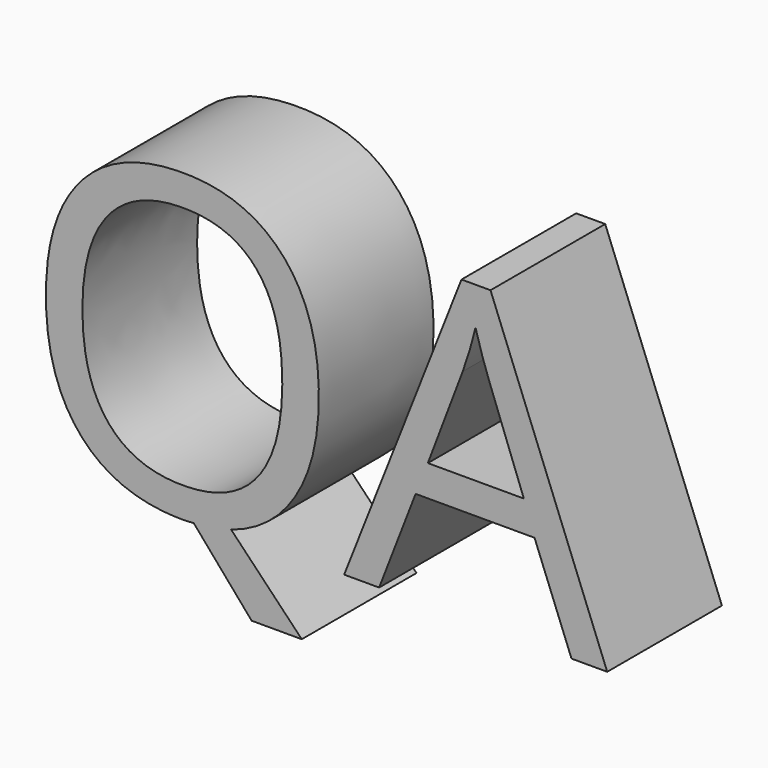
from build123d import *

# Parameters (mm, degrees)
F0_TEXT_SIZE = 107.5041739063
F1_DEPTH     = 37.084


# Not quite as in the source:
# - Text() gives the source's letters only with a copy of the font that has no kerning and outlines rounded to 1/6400 em; it was checked with that copy


with BuildPart() as f1:
    # F0 (on Front) → F1 (new body)
    with BuildSketch(Plane.XZ):
        with Locations((-60.6834925711, -34.4058983028)):
            Text('QA', F0_TEXT_SIZE, font='Open Sans', text_align=(TextAlign.LEFT, TextAlign.BOTTOM))
    extrude(amount=-F1_DEPTH)


solid = f1.part
